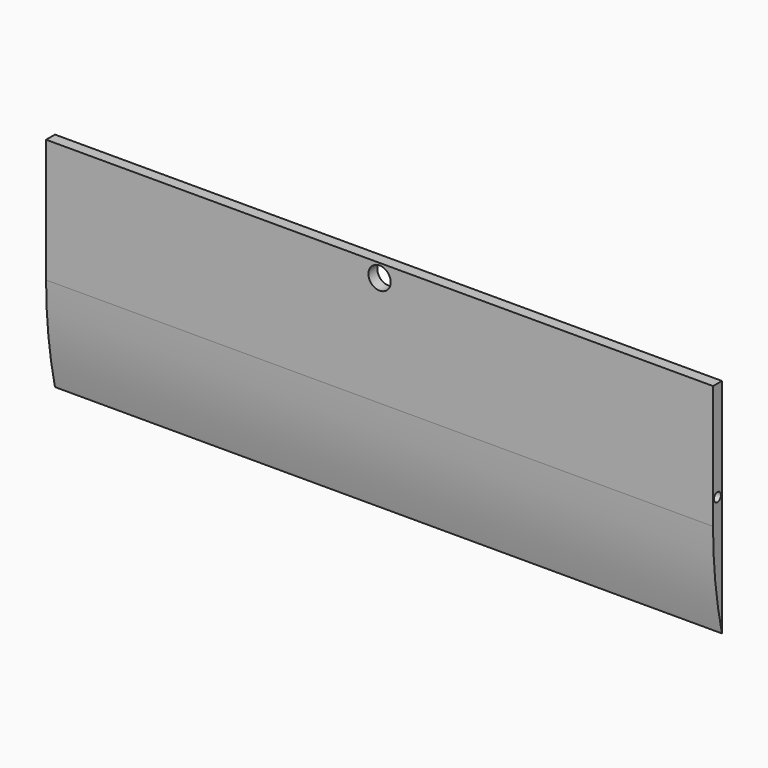
from build123d import *

# Parameters (mm, degrees)
F0_W        = 76.2
F0_H        = 25.4
F1_DEPTH    = 1.27
F2_T1_DEPTH = 132.64003455
F3_R        = 0.508
F4_DEPTH    = 1.27
F5_R        = 0.508
F6_DEPTH    = 1.27
F7_R        = 1.27
F8_DEPTH    = 25.4


# Not quite as in the source:
# - a fillet or chamfer that OpenCascade refuses, or shapes differently, is made with other operations: its cross-section is extruded or revolved along the edge and cut away or added


with BuildPart() as f1:
    # F0 (on Front) → F1 (new body)
    with BuildSketch(Plane.XZ):
        with Locations((-28.6749217987, 43.1045838744)):
            Rectangle(F0_W, F0_H)
    extrude(amount=F1_DEPTH)

    # F2: fillet of radius 50.8 on 1 edges, made by hand

    # F2_s2 → F2_t1 (cut)
    with BuildSketch(Plane.YZ.offset(-94.9949390737)):
        with BuildLine():
            ThreePointArc((0, 30.4045838744), (-0.9515015625, 36.0129781215), (-1.27, 41.6925907843))
            Line((-1.27, 41.6925907843), (-2.286, 41.6925907843))
            Line((-2.286, 41.6925907843), (-2.286, 30.4045838744))
            Line((-2.286, 30.4045838744), (-1.27, 29.3885838744))
            ThreePointArc((-1.27, 29.3885838744), (-0.635, 29.3885838744), (-0.9906, 30.1788237362))
            Line((-0.9906, 30.1788237362), (0, 30.4045838744))
        make_face()
    extrude(amount=F2_T1_DEPTH, mode=Mode.SUBTRACT)

    # F3 (on face) → F4 (cut)
    with BuildSketch(Plane(origin=(-66.7749217987, 0, 0), x_dir=(0, -1, 0), z_dir=(-1, 0, 0))):
        with Locations((0.635, 44.3745838744)):
            Circle(F3_R)
    extrude(amount=-F4_DEPTH, mode=Mode.SUBTRACT)

    # F5 (on face) → F6 (cut)
    with BuildSketch(Plane.YZ.offset(9.4250782013)):
        with Locations((-0.635, 44.3745838744)):
            Circle(F5_R)
    extrude(amount=-F6_DEPTH, mode=Mode.SUBTRACT)

    # F7 (on face) → F8 (cut)
    with BuildSketch(Plane.XZ.offset(1.27)):
        with Locations((-28.6749217987, 54.2805838744)):
            Circle(F7_R)
    extrude(amount=-F8_DEPTH, mode=Mode.SUBTRACT)


solid = f1.part
